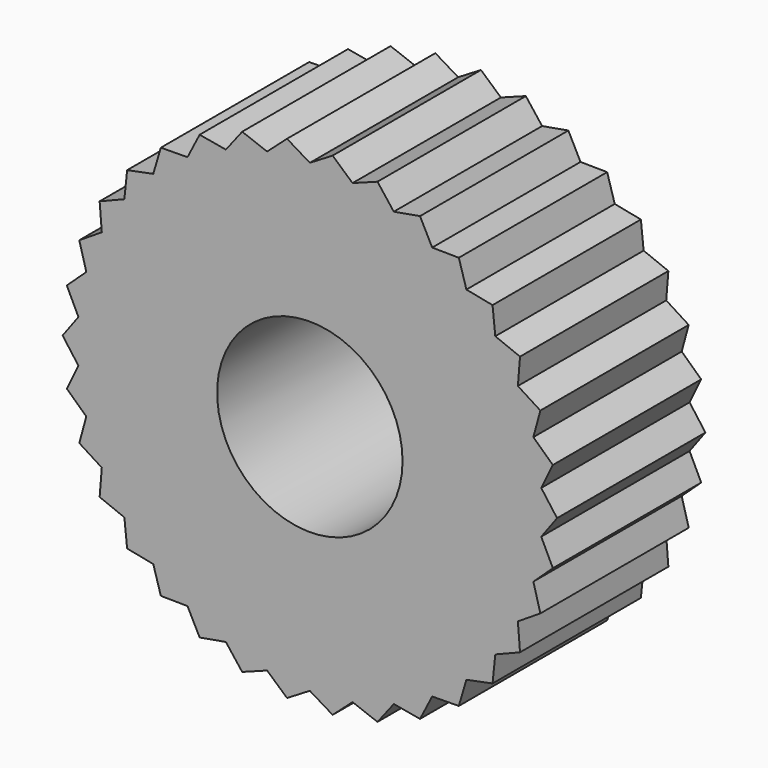
from build123d import *

# Parameters (mm, degrees)
F0_R            = 6.35
F0_R_2          = 2.38125
F1_DEPTH        = 4.7625
F3_DEPTH        = 4.7635
F3_COPIES_COUNT = 34


# Not quite as in the source:
# - a pattern or mirror of a feature is missing from the dataset's text; its kind, count and spacing are read off the source's solid


with BuildPart() as f1:
    # F0 (on Front) → F1 (new body)
    with BuildSketch(Plane.XZ):
        Circle(F0_R)
        Circle(F0_R_2, mode=Mode.SUBTRACT)
    extrude(amount=F1_DEPTH)

    # F2 (on Front) → F3 (cut, through all)
    with BuildSketch(Plane.XZ):
        with BuildLine():
            Line((-0.5859040826, 6.3229120195), (0, 5.969))
            Line((0, 5.969), (0.5859040826, 6.3229120195))
            ThreePointArc((0.5859040826, 6.3229120195), (0, 6.4661394577), (-0.5859040826, 6.3229120195))
        make_face()
    f3 = extrude(amount=F3_DEPTH, mode=Mode.SUBTRACT)

    # F3_copies: F3 ×34 about axis
    f3_copies_axis = Axis((0, 0, 0), (0, 1, 0))
    for i in range(1, F3_COPIES_COUNT):
        add(f3.rotate(f3_copies_axis, i * 360 / F3_COPIES_COUNT), mode=Mode.SUBTRACT)


solid = f1.part
